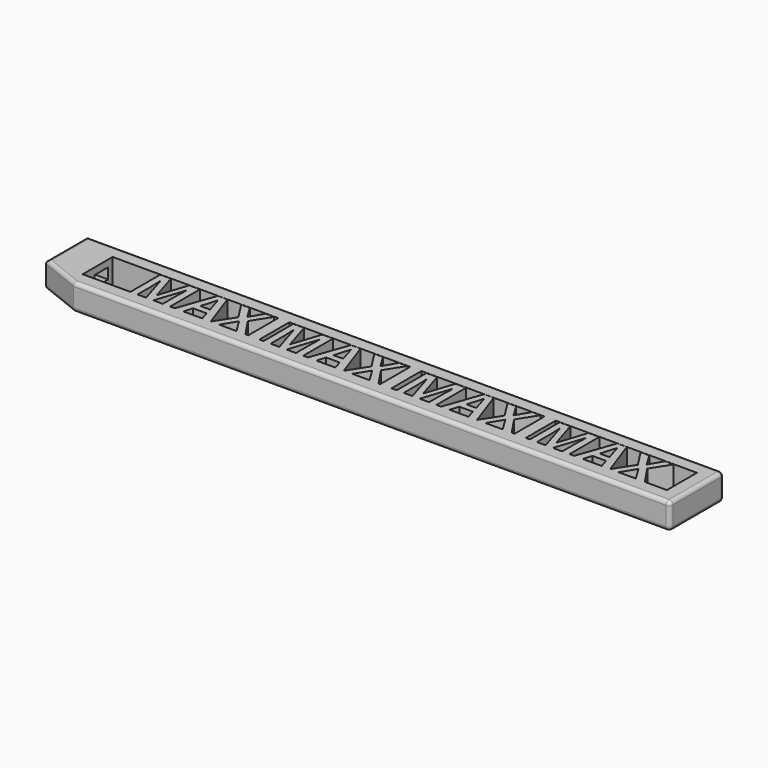
from build123d import *

# Parameters (mm, degrees)
F0_W          = 170
F0_H          = 18
F0_TEXT_SIZE  = 13.8888888889
F0_W_2        = 3
F0_H_2        = 10
F1_DEPTH      = 3.5
F3_DEPTH      = 1.7
F3_DEPTH_BACK = 1.2
F5_DEPTH      = 7.5
F6_R          = 1


# Not quite as in the source:
# - Text() gives the source's letters only with a copy of the font that has no kerning and outlines rounded to 1/6400 em; it was checked with that copy


with BuildPart() as f1:
    # F0 (on Top) → F1 (new body, symmetric)
    with BuildSketch(Plane.XY):
        with Locations((-30.7142301194, 0)):
            Rectangle(F0_W, F0_H)
        Polygon((-105.7142301194, -5), (-105.7142301194, 5), (-61.5231520295, 5), (-58.5231520295, 5), (-26.2669644944, 5), (-23.2669644944, 5), (9.5946029961, 5), (12.5946029961, 5), (50.2857698806, 5), (50.2857698806, -5), (44.3851622417, -5), (41.9849886306, -5), (37.3734434917, -5), (35.120839325, -5), (32.855214325, -5), (27.8031309917, -5), (25.5375059917, -5), (24.2896761306, -5), (22.3300407139, -5), (19.8148497417, -5), (17.8877664084, -5), (15.570058075, -5), (13.6907177972, -5), (12.5946029961, -5), (9.5946029961, -5), (8.8339469639, -5), (6.4337733528, -5), (1.8222282139, -5), (-0.4303759528, -5), (-2.6960009528, -5), (-7.7480842861, -5), (-10.0137092861, -5), (-11.2615391472, -5), (-13.2211745639, -5), (-15.7363655361, -5), (-17.6634488694, -5), (-19.9811572028, -5), (-21.8604974805, -5), (-23.2669644944, -5), (-26.2669644944, -5), (-26.7172683139, -5), (-29.117441925, -5), (-33.7289870639, -5), (-35.9815912305, -5), (-38.2472162305, -5), (-43.2992995639, -5), (-45.5649245639, -5), (-46.812754425, -5), (-48.7723898416, -5), (-51.2875808139, -5), (-53.2146641472, -5), (-55.5323724805, -5), (-57.4117127583, -5), (-58.5231520295, -5), (-61.5231520295, -5), (-62.2684835916, -5), (-64.6686572028, -5), (-69.2802023416, -5), (-71.5328065083, -5), (-73.7984315083, -5), (-78.8505148416, -5), (-81.1161398416, -5), (-82.3639697028, -5), (-84.3236051194, -5), (-86.8387960916, -5), (-88.765879425, -5), (-91.0835877583, -5), (-92.9629280361, -5), align=None, mode=Mode.SUBTRACT)
        with Locations((-94.2107578972, -5)):
            Text('MAX MAX MAX MAX', F0_TEXT_SIZE, font='Open Sans', font_style=FontStyle.BOLD, text_align=(TextAlign.LEFT, TextAlign.BOTTOM))
        with Locations((-60.0231520295, 0)):
            Rectangle(F0_W_2, F0_H_2)
        with Locations((-24.7669644944, 0)):
            Rectangle(F0_W_2, F0_H_2)
        with Locations((11.0946029961, 0)):
            Rectangle(F0_W_2, F0_H_2)
    extrude(amount=F1_DEPTH, both=True)

    # F2 (on Top) → F3 (cut, two sides)
    with BuildSketch(Plane.XY) as f3_sk:
        Polygon((-105.2142301194, 3.5), (-116.7142301194, 3.5), (-116.7142301194, -2.5), (-105.2142301194, -1), align=None)
    extrude(amount=F3_DEPTH, mode=Mode.SUBTRACT)
    extrude(f3_sk.sketch, amount=-F3_DEPTH_BACK, mode=Mode.SUBTRACT)

    # F4 (on Top) → F5 (cut, symmetric)
    with BuildSketch(Plane.XY):
        Polygon((-117.7709698677, -10.5618461967), (-104.4237911701, -9.2072207481), (-117.7709698677, -3.8991386537), align=None)
    extrude(amount=F5_DEPTH, both=True, mode=Mode.SUBTRACT)

    # F6
    f6_edges = [f1.edges().sort_by_distance(p)[0] for p in [
        (54.28577, 0, -3.5),
        (-30.71423, 9, -3.5),
        (-25.329539, -9, -3.5),
        (54.28577, 0, 3.5),
        (54.28577, 9, 0),
        (54.28577, -9, 0),
        (-110.329539, -6.858545, -3.5),
        (-25.329539, -9, 3.5),
        (-30.71423, 9, 3.5),
        (-115.71423, 2.141455, 3.5),
        (-110.329539, -6.858545, 3.5),
    ]]
    fillet(f6_edges, radius=F6_R)


solid = f1.part
